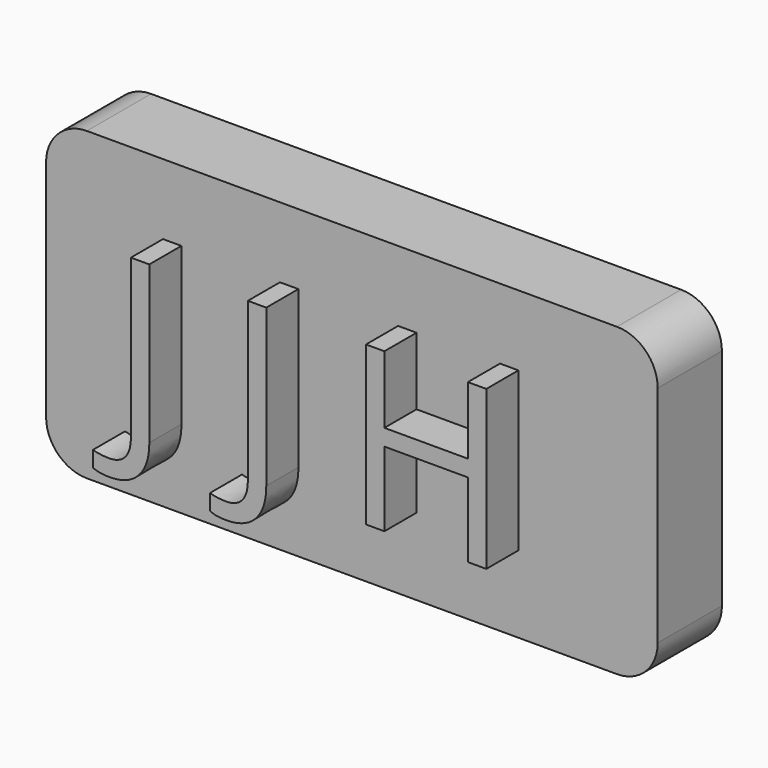
from build123d import *

# Parameters (mm, degrees)
F0_W         = 76.2
F0_H         = 38.1
F1_DEPTH     = 10
F2_TEXT_SIZE = 27.6556651922
F3_DEPTH     = 5
F4_TEXT_SIZE = 21.2520179856
F5_DEPTH     = 5
F6_R         = 5.08


# Not quite as in the source:
# - Text() gives the source's letters only with a copy of the font that has no kerning and outlines rounded to 1/6400 em; it was checked with that copy


with BuildPart() as f1:
    # F0 (on Front) → F1 (new body)
    with BuildSketch(Plane.XZ):
        with Locations((38.1, 19.05)):
            Rectangle(F0_W, F0_H)
    extrude(amount=F1_DEPTH)

    # F2 (on face) → F3 (join)
    with BuildSketch(Plane.XZ.offset(10)):
        with Locations((11.9995431792, 9.5811236802)):
            Text('J J H', F2_TEXT_SIZE, font='Open Sans', text_align=(TextAlign.LEFT, TextAlign.BOTTOM))
    extrude(amount=F3_DEPTH)

    # F4 (on face) → F5 (join)
    with BuildSketch(Plane(origin=(0, 0, 0), x_dir=(-1, 0, 0), z_dir=(0, 1, 0))):
        with Locations((-62.7728160471, 11.5221776068)):
            Text('Meta', F4_TEXT_SIZE, font='Open Sans', text_align=(TextAlign.LEFT, TextAlign.BOTTOM))
    extrude(amount=F5_DEPTH)

    # F6
    f6_edges = [f1.edges().sort_by_distance(p)[0] for p in [
        (0, -5, 38.1),
        (0, -5, 0),
        (76.2, -5, 0),
        (76.2, -5, 38.1),
    ]]
    fillet(f6_edges, radius=F6_R)


solid = f1.part
